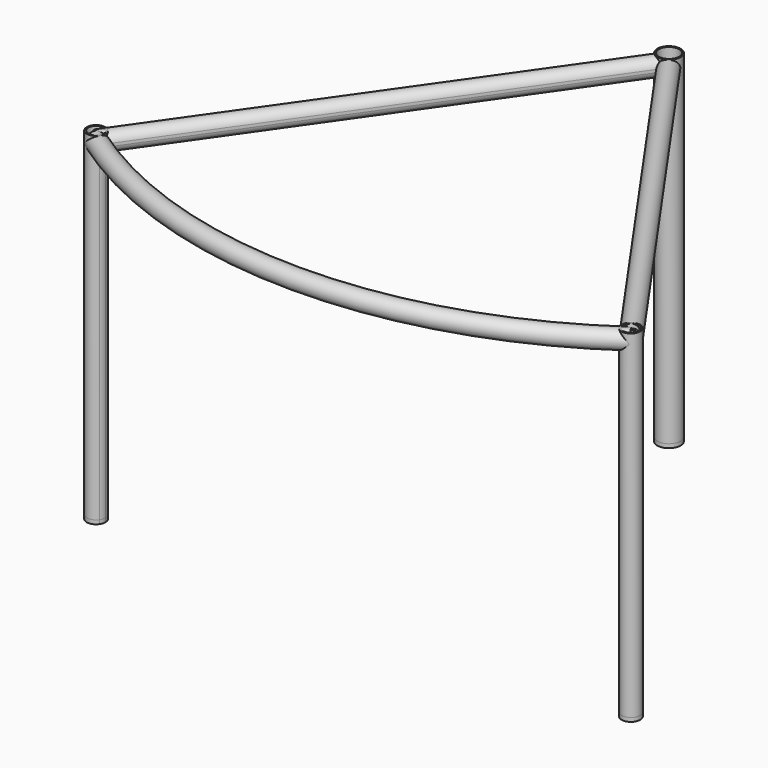
from build123d import *

# Parameters (mm, degrees)
F0_W     = 220
F0_H     = 220
F1_DEPTH = 3
F3_R     = 75
F3_R_2   = 65
F4_DEPTH = 2200
F5_DEPTH = 25
F8_R     = 50
F9_REACH = 4251.7766190325
F12_R    = 60
F12_R_2  = 50


with BuildPart() as f1:
    # F0 (on Front) → F1 (new body)
    with BuildSketch(Plane.XZ):
        Rectangle(F0_W, F0_H)
    extrude(amount=F1_DEPTH)


with BuildPart() as f4:
    # F3 (on Top) → F4 (new body)
    with BuildSketch(Plane.XY):
        Circle(F3_R)
        Circle(F3_R_2, mode=Mode.SUBTRACT)
    extrude(amount=F4_DEPTH)


with BuildPart() as f4b:
    # F3 (on Top) → F4, piece 2 (new body)
    with BuildSketch(Plane.XY):
        with BuildLine():
            ThreePointArc((-1660.7293090531, -2457.456132867), (-1778.0418236555, -2439.7001290949), (-1671.2384980516, -2491.3775070491))
            ThreePointArc((-1671.2384980516, -2491.3775070491), (-1663.4167944508, -2475.212136639), (-1660.7293090531, -2457.456132867))
        make_face()
        with BuildLine():
            ThreePointArc((-1670.7293090531, -2457.456132867), (-1672.981227879, -2472.2925995685), (-1679.5341388205, -2485.792645523))
            ThreePointArc((-1679.5341388205, -2485.792645523), (-1768.4773902273, -2442.6196661655), (-1670.7293090531, -2457.456132867))
        make_face(mode=Mode.SUBTRACT)
    extrude(amount=F4_DEPTH)


with BuildPart() as f4c:
    # F3 (on Top) → F4, piece 3 (new body)
    with BuildSketch(Plane.XY):
        with BuildLine():
            ThreePointArc((1780.7293090531, -2457.456132867), (1702.9733052811, -2400.1436182646), (1671.2384980516, -2491.3775070491))
            ThreePointArc((1671.2384980516, -2491.3775070491), (1738.4853128252, -2514.7686474693), (1780.7293090531, -2457.456132867))
        make_face()
        with BuildLine():
            ThreePointArc((1770.7293090531, -2457.456132867), (1735.5657757546, -2505.2042140411), (1679.5341388205, -2485.792645523))
            ThreePointArc((1679.5341388205, -2485.792645523), (1705.8928423516, -2409.7080516928), (1770.7293090531, -2457.456132867))
        make_face(mode=Mode.SUBTRACT)
    extrude(amount=F4_DEPTH)


with BuildPart() as f5:
    # F3 (on Top) → F5 (new body)
    with BuildSketch(Plane.XY):
        Circle(F3_R)
        Circle(F3_R_2, mode=Mode.SUBTRACT)
    extrude(amount=F5_DEPTH)


with BuildPart() as f5b:
    # F3 (on Top) → F5, piece 2 (new body)
    with BuildSketch(Plane.XY):
        with BuildLine():
            ThreePointArc((-1660.7293090531, -2457.456132867), (-1778.0418236555, -2439.7001290949), (-1671.2384980516, -2491.3775070491))
            ThreePointArc((-1671.2384980516, -2491.3775070491), (-1663.4167944508, -2475.212136639), (-1660.7293090531, -2457.456132867))
        make_face()
        with BuildLine():
            ThreePointArc((-1670.7293090531, -2457.456132867), (-1672.981227879, -2472.2925995685), (-1679.5341388205, -2485.792645523))
            ThreePointArc((-1679.5341388205, -2485.792645523), (-1768.4773902273, -2442.6196661655), (-1670.7293090531, -2457.456132867))
        make_face(mode=Mode.SUBTRACT)
    extrude(amount=F5_DEPTH)


with BuildPart() as f5c:
    # F3 (on Top) → F5, piece 3 (new body)
    with BuildSketch(Plane.XY):
        with BuildLine():
            ThreePointArc((1780.7293090531, -2457.456132867), (1702.9733052811, -2400.1436182646), (1671.2384980516, -2491.3775070491))
            ThreePointArc((1671.2384980516, -2491.3775070491), (1738.4853128252, -2514.7686474693), (1780.7293090531, -2457.456132867))
        make_face()
        with BuildLine():
            ThreePointArc((1770.7293090531, -2457.456132867), (1735.5657757546, -2505.2042140411), (1679.5341388205, -2485.792645523))
            ThreePointArc((1679.5341388205, -2485.792645523), (1705.8928423516, -2409.7080516928), (1770.7293090531, -2457.456132867))
        make_face(mode=Mode.SUBTRACT)
    extrude(amount=F5_DEPTH)


with BuildPart() as f9:
    f9_end = f4.part.faces().sort_by_distance((-75, 0, 1100))[0]
    # F8 (on line) → F9 (new body, up to a face of F4 that its end follows)
    with BuildSketch(Plane(origin=(-1720.7293090531, -2457.456132867, 0), x_dir=(0.8191520443, -0.5735764364, 0), z_dir=(-0.5735764364, -0.8191520443, 0))):
        with BuildLine():
            ThreePointArc((59.2933781445, 2148.8258439111), (-4.6041997855, 2199.4676799799), (-60, 2139.6445962719))
            ThreePointArc((-60, 2139.6445962719), (-44.6724411369, 2099.589971035), (-6.5208999043, 2080))
            Line((-6.5208999043, 2080), (6.5208999043, 2080))
            ThreePointArc((6.5208999043, 2080), (41.4670614775, 2096.2800622329), (59.2933781445, 2130.4633486327))
            Line((59.2933781445, 2130.4633486327), (59.2933781445, 2148.8258439111))
        make_face()
        with Locations((0, 2139.6445962719)):
            Circle(F8_R, mode=Mode.SUBTRACT)
    f9_long = extrude(amount=-F9_REACH, mode=Mode.PRIVATE)
    add(split(f9_long, bisect_by=f9_end, keep=Keep.ALL, mode=Mode.PRIVATE).solids().sort_by_distance((-1755.2511826319, -2433.283656754, 2179.9439809286))[0])


with BuildPart() as f10_1:
    # F10: instance of F9
    add(f9.part.mirror(Plane.YZ))


with BuildPart() as f13:
    # F13: sweep along a path in F11
    with BuildLine(Plane.XY.offset(2200)) as f13_path:
        ThreePointArc((-1720.7293090531, -2457.456132867), (0, -3000), (1720.7293090531, -2457.456132867))
    # F12 (on Right) → F13 (sweep)
    with BuildSketch(Plane.YZ):
        with Locations((-3000, 2140)):
            Circle(F12_R)
        with Locations((-3000, 2140)):
            Circle(F12_R_2, mode=Mode.SUBTRACT)
    sweep(path=f13_path.line)


solid = Compound([f4.part, f4b.part, f4c.part, f5.part, f5b.part, f5c.part, f9.part, f10_1.part, f13.part])
